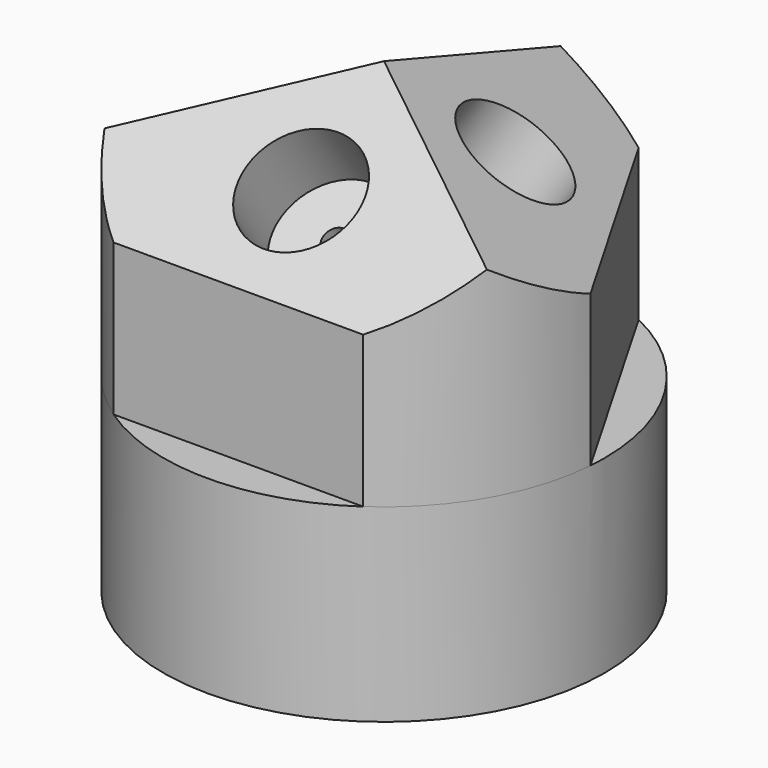
from build123d import *

# Parameters (mm, degrees)
F3_DEPTH       = 12
F8_R           = 1
F9_DEPTH       = 8
F10_R          = 4.5
F11_DEPTH      = 2
F12_R          = 1
F13_REACH      = 37.3532145158
F12_R_2        = 4.5
F14_DEPTH      = 6
F16_END_RADIUS = 1
F15_R          = 1
F16_REACH      = 37.3532145367
F15_R_2        = 4.5
F17_DEPTH      = 6
F19_END_RADIUS = 1
F18_R          = 1
F19_REACH      = 37.3532145367
F18_R_2        = 4.5
F20_DEPTH      = 6
F22_DEPTH      = 25
F23_R          = 17.5
F23_R_2        = 1.5
F23_R_3        = 6.5
F23_R_4        = 4.5
F24_DEPTH      = 15
F25_DEPTH      = 10


with BuildPart() as f3:
    # F2 (on Top) → F3 (new body)
    with BuildSketch(Plane.XY):
        Polygon((25, -14.4337567297), (0, 28.8675134595), (-25, -14.4337567297), align=None)
    extrude(amount=-F3_DEPTH)

    # F3_face (on face) → F6 section 0
    with BuildSketch(Plane.XY, mode=Mode.PRIVATE) as f6_s0:
        Polygon((-25, -14.4337567297), (25, -14.4337567297), (0, 28.8675134595), align=None)
    loft([f6_s0.sketch, Vertex(0, 0, 10)])

    # F8 (on face) → F9 (cut)
    with BuildSketch(Plane(origin=(0, 0, -12), x_dir=(1, 0, 0), z_dir=(0, 0, -1))):
        Circle(F8_R)
    extrude(amount=-F9_DEPTH, mode=Mode.SUBTRACT)

    # F10 (on face) → F11 (cut)
    with BuildSketch(Plane(origin=(0, 0, -12), x_dir=(1, 0, 0), z_dir=(0, 0, -1))):
        Circle(F10_R)
    extrude(amount=-F11_DEPTH, mode=Mode.SUBTRACT)

    f13_end = f3.faces().sort_by_distance((-1, 0, -7))[0]
    # F12 (on face) → F13 (cut, up to a face of the model that its end follows)
    with BuildSketch(Plane(origin=(0, -4.6812183988, 6.7567567568), x_dir=(1, 0, 0), z_dir=(0, -0.5694947975, 0.8219949365))):
        with Locations((0, -4.3050520255)):
            Circle(F12_R)
    f13_long = extrude(amount=-F13_REACH, mode=Mode.PRIVATE)
    add(split(f13_long, bisect_by=f13_end, keep=Keep.BOTTOM, mode=Mode.PRIVATE), mode=Mode.SUBTRACT)

    # F12 (on face) → F14 (cut)
    with BuildSketch(Plane(origin=(0, -4.6812183988, 6.7567567568), x_dir=(1, 0, 0), z_dir=(0, -0.5694947975, 0.8219949365))):
        with Locations((0, -4.3050520255)):
            Circle(F12_R_2)
        with Locations((0, -4.3050520255)):
            Circle(F12_R, mode=Mode.SUBTRACT)
    extrude(amount=-F14_DEPTH, mode=Mode.SUBTRACT)

    f16_end = (Plane(origin=(0, 0, -7), x_dir=(-1, 0, 0), z_dir=(0, 0, -1)) * Cylinder(F16_END_RADIUS, 214.1194850146, mode=Mode.PRIVATE)).faces().sort_by_distance((-1, 0, -7))[0]
    # F15 (on face) → F16 (cut, up to the whole of a round face its end follows)
    with BuildSketch(Plane(origin=(-4.0540540541, 2.3406091994, 6.7567567568), x_dir=(0.8699176724, 0.1614366008, 0.4660273245), z_dir=(-0.4931969619, 0.2847473987, 0.8219949365))):
        with Locations((-3.5228976388, 2.474401982)):
            Circle(F15_R)
    f16_long = extrude(amount=-F16_REACH, mode=Mode.PRIVATE)
    add(split(f16_long, bisect_by=f16_end, keep=Keep.ALL, mode=Mode.PRIVATE).solids().sort_by_distance((-7.1186849681, 4.1099746826, 4.3050520255))[0], mode=Mode.SUBTRACT)

    # F15 (on face) → F17 (cut)
    with BuildSketch(Plane(origin=(-4.0540540541, 2.3406091994, 6.7567567568), x_dir=(0.8699176724, 0.1614366008, 0.4660273245), z_dir=(-0.4931969619, 0.2847473987, 0.8219949365))):
        with Locations((-3.5228976388, 2.474401982)):
            Circle(F15_R_2)
        with Locations((-3.5228976388, 2.474401982)):
            Circle(F15_R, mode=Mode.SUBTRACT)
    extrude(amount=-F17_DEPTH, mode=Mode.SUBTRACT)

    f19_end = (Plane(origin=(0, 0, -7), x_dir=(-1, 0, 0), z_dir=(0, 0, -1)) * Cylinder(F19_END_RADIUS, 214.1194850146, mode=Mode.PRIVATE)).faces().sort_by_distance((-1, 0, -9.9336675042))[0]
    # F18 (on face) → F19 (cut, up to the whole of a round face its end follows)
    with BuildSketch(Plane(origin=(4.0540540541, 2.3406091994, 6.7567567568), x_dir=(0.8699176724, -0.1614366008, -0.4660273245), z_dir=(0.4931969619, 0.2847473987, 0.8219949365))):
        with Locations((3.5228976388, 2.474401982)):
            Circle(F18_R)
    f19_long = extrude(amount=-F19_REACH, mode=Mode.PRIVATE)
    add(split(f19_long, bisect_by=f19_end, keep=Keep.ALL, mode=Mode.PRIVATE).solids().sort_by_distance((7.1186849681, 4.1099746826, 4.3050520255))[0], mode=Mode.SUBTRACT)

    # F18 (on face) → F20 (cut)
    with BuildSketch(Plane(origin=(4.0540540541, 2.3406091994, 6.7567567568), x_dir=(0.8699176724, -0.1614366008, -0.4660273245), z_dir=(0.4931969619, 0.2847473987, 0.8219949365))):
        with Locations((3.5228976388, 2.474401982)):
            Circle(F18_R_2)
        with Locations((3.5228976388, 2.474401982)):
            Circle(F18_R, mode=Mode.SUBTRACT)
    extrude(amount=-F20_DEPTH, mode=Mode.SUBTRACT)

    # F21 (on face) → F22 (cut)
    with BuildSketch(Plane(origin=(0, 0, -12), x_dir=(1, 0, 0), z_dir=(0, 0, -1))):
        with BuildLine():
            Line((3.2541491538, -23.2311617897), (7.5523574637, -15.7864466154))
            ThreePointArc((7.5523574637, -15.7864466154), (0, -17.5), (-7.5523574637, -15.7864466154))
            Line((-7.5523574637, -15.7864466154), (-3.2541491538, -23.2311617897))
            ThreePointArc((-3.2541491538, -23.2311617897), (0, -23.4579701768), (3.2541491538, -23.2311617897))
        make_face()
        with BuildLine():
            ThreePointArc((-9.8952850725, 14.4337567297), (0, 17.5), (9.8952850725, 14.4337567297))
            Line((9.8952850725, 14.4337567297), (18.4917016925, 14.4337567297))
            ThreePointArc((18.4917016925, 14.4337567297), (0, 23.4579701768), (-18.4917016925, 14.4337567297))
            Line((-18.4917016925, 14.4337567297), (-9.8952850725, 14.4337567297))
        make_face()
        with BuildLine():
            ThreePointArc((-17.4476425363, 1.3526898856), (-15.1554445662, 8.75), (-9.8952850725, 14.4337567297))
            Line((-9.8952850725, 14.4337567297), (-18.4917016925, 14.4337567297))
            ThreePointArc((-18.4917016925, 14.4337567297), (-20.3151980943, 11.7289850884), (-21.7458508462, 8.79740506))
            Line((-21.7458508462, 8.79740506), (-17.4476425363, 1.3526898856))
        make_face()
        with BuildLine():
            ThreePointArc((9.8952850725, 14.4337567297), (15.1554445662, 8.75), (17.4476425363, 1.3526898856))
            Line((17.4476425363, 1.3526898856), (21.7458508462, 8.79740506))
            ThreePointArc((21.7458508462, 8.79740506), (20.3151980943, 11.7289850884), (18.4917016925, 14.4337567297))
            Line((18.4917016925, 14.4337567297), (9.8952850725, 14.4337567297))
        make_face()
        with BuildLine():
            Line((0, -28.8675134595), (3.2541491538, -23.2311617897))
            ThreePointArc((3.2541491538, -23.2311617897), (0, -23.4579701768), (-3.2541491538, -23.2311617897))
            Line((-3.2541491538, -23.2311617897), (0, -28.8675134595))
        make_face()
        with BuildLine():
            ThreePointArc((-21.7458508462, 8.79740506), (-20.3151980943, 11.7289850884), (-18.4917016925, 14.4337567297))
            Line((-18.4917016925, 14.4337567297), (-25, 14.4337567297))
            Line((-25, 14.4337567297), (-21.7458508462, 8.79740506))
        make_face()
        with BuildLine():
            ThreePointArc((18.4917016925, 14.4337567297), (20.3151980943, 11.7289850884), (21.7458508462, 8.79740506))
            Line((21.7458508462, 8.79740506), (25, 14.4337567297))
            Line((25, 14.4337567297), (18.4917016925, 14.4337567297))
        make_face()
    extrude(amount=-F22_DEPTH, mode=Mode.SUBTRACT)

    # F23 (on face) → F24 (join)
    with BuildSketch(Plane(origin=(0, 0, -12), x_dir=(1, 0, 0), z_dir=(0, 0, -1))):
        Circle(F23_R)
        with Locations((-10.8253175473, -6.25)):
            Circle(F23_R_2, mode=Mode.SUBTRACT)
        Circle(F23_R_3, mode=Mode.SUBTRACT)
        with Locations((10.8253175473, 6.25)):
            Circle(F23_R_2, mode=Mode.SUBTRACT)
        Circle(F23_R_3)
        Circle(F23_R_4, mode=Mode.SUBTRACT)
    extrude(amount=F24_DEPTH)

    # F25 (add): a face of the model
    f25_faces = [f3.faces().sort_by_distance(p)[0] for p in [
        (-4.3727207794, 0, -10),
    ]]
    extrude(f25_faces, amount=F25_DEPTH)


solid = f3.part
